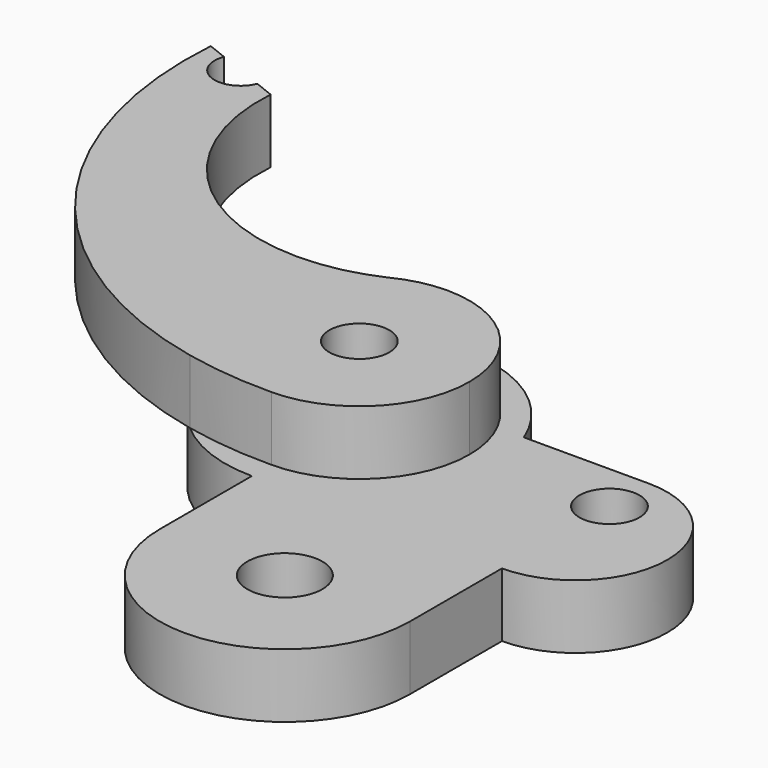
from build123d import *

# Parameters (mm, degrees)
F0_R     = 1.875
F0_R_2   = 5.5
F1_DEPTH = 3.2
F3_R     = 1.5
F4_DEPTH = 3.2
F2_R     = 1.5
F5_DEPTH = 3.2


with BuildPart() as f1:
    # F0 (on Top) → F1 (new body)
    with BuildSketch(Plane.XY):
        with BuildLine():
            ThreePointArc((-6.25, 19.187701866), (-12.968850933, 12.468850933), (-6.25, 5.75))
            Line((-6.25, 5.75), (-6.25, 0))
            ThreePointArc((-6.25, 0), (0, -6.25), (6.25, 0))
            Line((6.25, 0), (6.25, 5.75))
            ThreePointArc((6.25, 5.75), (10.8423546879, 10.3423546879), (6.25, 14.9347093758))
            Line((6.25, 14.9347093758), (0, 14.9347093758))
            ThreePointArc((0, 14.9347093758), (-2.4701043294, 18.0236098458), (-6.25, 19.187701866))
        make_face()
        Circle(F0_R, mode=Mode.SUBTRACT)
        with Locations((-6.25, 12.468850933)):
            Circle(F0_R_2, mode=Mode.SUBTRACT)
    extrude(amount=F1_DEPTH)

    # F2 (on face) → F5 (cut, through all)
    with BuildSketch(Plane.XY.offset(3.2)):
        with Locations((6.25, 12.468850933)):
            Circle(F2_R)
    extrude(amount=-F5_DEPTH, mode=Mode.SUBTRACT)


with BuildPart() as f4:
    # F3 (on face) → F4 (new body)
    with BuildSketch(Plane.XY.offset(3.2)):
        with BuildLine():
            ThreePointArc((-8.7732377369, 17.3559023265), (-11.5945665243, 11.1705410055), (-6.25, 6.968850933))
            ThreePointArc((-6.25, 6.968850933), (-2.3609127035, 8.5797636365), (-0.75, 12.468850933))
            ThreePointArc((-0.75, 12.468850933), (-3.388864522, 17.1660739186), (-8.7732377369, 17.3559023265))
        make_face()
        with Locations((-6.25, 12.468850933)):
            Circle(F3_R, mode=Mode.SUBTRACT)
        with BuildLine():
            ThreePointArc((-10.6767033745, 7.4144216779), (-8.4758217458, 7.0677474483), (-6.25, 6.968850933))
            ThreePointArc((-6.25, 6.968850933), (-11.5945665243, 11.1705410055), (-8.7732377369, 17.3559023265))
            ThreePointArc((-8.7732377369, 17.3559023265), (-10.1339419751, 16.8675420062), (-11.5534928512, 16.5938868646))
            ThreePointArc((-11.5534928512, 16.5938868646), (-12.9384097457, 11.8299981064), (-10.6767033745, 7.4144216779))
        make_face()
        with BuildLine():
            ThreePointArc((-26.3622067869, 28.3246971667), (-22.4253559313, 14.9396113614), (-10.6767033745, 7.4144216779))
            ThreePointArc((-10.6767033745, 7.4144216779), (-12.9384097457, 11.8299981064), (-11.5534928512, 16.5938868646))
            ThreePointArc((-11.5534928512, 16.5938868646), (-19.1117610171, 19.1441645492), (-21.9799764454, 26.5875961632))
            Line((-21.9799764454, 26.5875961632), (-22.9542631916, 26.9738000713))
            ThreePointArc((-22.9542631916, 26.9738000713), (-24.6534382097, 26.2393182404), (-25.3879200407, 27.9384932585))
            Line((-25.3879200407, 27.9384932585), (-26.3622067869, 28.3246971667))
        make_face()
    extrude(amount=F4_DEPTH)


solid = Compound([f1.part, f4.part])
